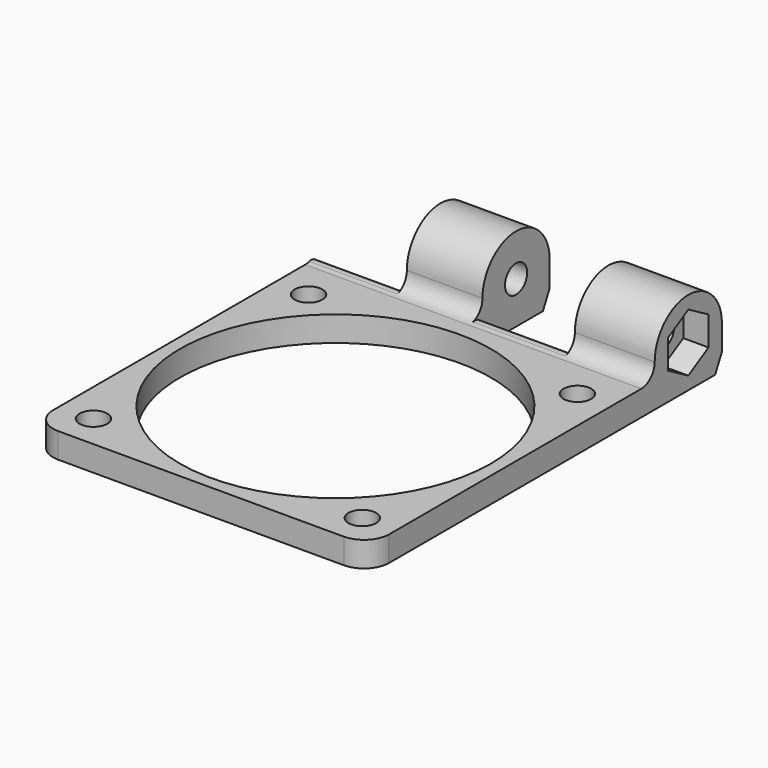
from build123d import *

# Parameters (mm, degrees)
F0_R      = 1.65
F0_R_2    = 18.5
F1_DEPTH  = 3
F3_DEPTH  = 40
F4_R      = 1.65
F5_DEPTH  = 40.001
F7_DEPTH  = 3
F8_R      = 1.99999
F11_DEPTH = 11
F14_DEPTH = 10.501
F15_SIZE2 = 2
F15_SIZE  = 1
F16_R     = 1


# Not quite as in the source:
# - a fillet or chamfer is up to 0.001 mm smaller than in the source, because OpenCascade refuses the exact size


with BuildPart() as f1:
    # F0 (on Top) → F1 (new body)
    with BuildSketch(Plane.XY):
        with BuildLine():
            Line((40, 0), (0, 0))
            Line((0, 0), (0, -42))
            ThreePointArc((0, -42), (0.8786796564, -44.1213203436), (3, -45))
            Line((3, -45), (37, -45))
            ThreePointArc((37, -45), (39.1213203436, -44.1213203436), (40, -42))
            Line((40, -42), (40, 0))
        make_face()
        with Locations((4, -41)):
            Circle(F0_R, mode=Mode.SUBTRACT)
        with Locations((36, -41)):
            Circle(F0_R, mode=Mode.SUBTRACT)
        with Locations((20, -25)):
            Circle(F0_R_2, mode=Mode.SUBTRACT)
        with Locations((4, -9)):
            Circle(F0_R, mode=Mode.SUBTRACT)
        with Locations((36, -9)):
            Circle(F0_R, mode=Mode.SUBTRACT)
    extrude(amount=F1_DEPTH)

    # F2 (on Right) → F3 (join)
    with BuildSketch(Plane.YZ):
        with BuildLine():
            Line((-2.5, 5), (-2.5, 0))
            Line((-2.5, 0), (7.5, 0))
            Line((7.5, 0), (7.5, 5))
            ThreePointArc((7.5, 5), (2.5, 10), (-2.5, 5))
        make_face()
    extrude(amount=F3_DEPTH)

    # F4 (on face) → F5 (cut, through all)
    with BuildSketch(Plane.YZ.offset(40)):
        with Locations((2.5, 5)):
            Circle(F4_R)
    extrude(amount=-F5_DEPTH, mode=Mode.SUBTRACT)

    # F6 (on face) → F7 (cut)
    with BuildSketch(Plane.YZ.offset(40)):
        Polygon((5.5, 3.2679491924), (5.5, 6.7320508076), (2.5, 8.4641016151), (-0.5, 6.7320508076), (-0.5, 3.2679491924), (2.5, 1.5358983849), align=None)
    extrude(amount=-F7_DEPTH, mode=Mode.SUBTRACT)

    # F8 (radius 2 in the source; OpenCascade refuses exactly that, so slightly less here)
    f8_edges = [f1.edges().sort_by_distance(p)[0] for p in [
        (20, -2.5, 3),
    ]]
    fillet(f8_edges, radius=F8_R)

    # F10 (on offset) → F11 (cut)
    with BuildSketch(Plane.YZ.offset(30.5)):
        with BuildLine():
            Line((8.25, -0.75), (8.25, 5))
            ThreePointArc((8.25, 5), (-1.5658639918, 9.0658639918), (2.5, -0.75))
            Line((2.5, -0.75), (8.25, -0.75))
        make_face()
    extrude(amount=-F11_DEPTH, mode=Mode.SUBTRACT)

    # F13 (on offset) → F14 (cut, through all)
    with BuildSketch(Plane.YZ.offset(10.5)):
        with BuildLine():
            Line((8.25, -0.75), (8.25, 5))
            ThreePointArc((8.25, 5), (-1.5658639918, 9.0658639918), (2.5, -0.75))
            Line((2.5, -0.75), (8.25, -0.75))
        make_face()
    extrude(amount=-F14_DEPTH, mode=Mode.SUBTRACT)

    # F15
    f15_edges = [f1.edges().sort_by_distance(p)[0] for p in [
        (35.25, 7.5, 0),
        (15, 7.5, 0),
    ]]
    f15_side = f1.faces().sort_by_distance((15, 6.839981, 0))[0]
    chamfer(f15_edges, length=F15_SIZE, length2=F15_SIZE2, reference=f15_side)

    # F16
    f16_edges = [f1.edges().sort_by_distance(p)[0] for p in [
        (25, -3.075892, 3.595745),
        (25, -0.339454, 0),
        (5.25, -3.075892, 3.595745),
        (5.25, -0.339454, 0),
    ]]
    fillet(f16_edges, radius=F16_R)


solid = f1.part
